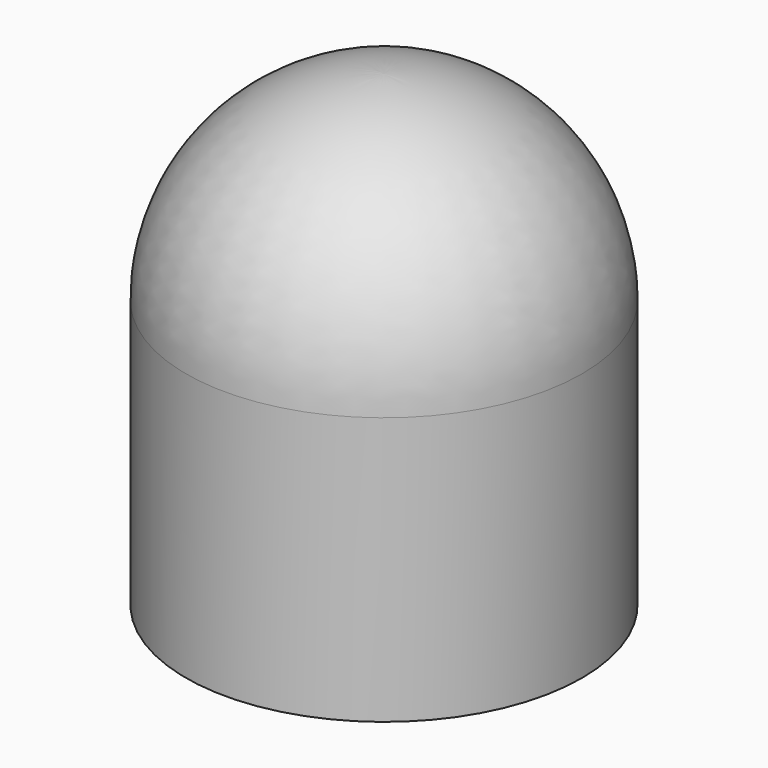
from build123d import *

# Parameters (mm, degrees)
F0_W = 0.381
F0_H = 7.3270857248


# Not quite as in the source:
# - a feature names something its author has since deleted; it is built from what else it names


with BuildPart() as f1:
    # F0 (on Front) → F1 (revolve)
    with BuildSketch(Plane.XZ):
        with BuildLine():
            ThreePointArc((0, 12.4069226423), (3.5657601658, 10.9047678598), (5.0392950625, 7.3270857248))
            Line((5.0392950625, 7.3270857248), (5.4202950625, 7.3270857248))
            ThreePointArc((5.4202950625, 7.3270857248), (3.8351698453, 11.1741775704), (0, 12.7879340205))
            Line((0, 12.7879340205), (0, 12.4069226423))
        make_face()
        with Locations((5.2297950625, 3.6635428624)):
            Rectangle(F0_W, F0_H)
    revolve(axis=Axis((0, 0, 8.3369510248), (0, 0, 1)))


solid = f1.part
